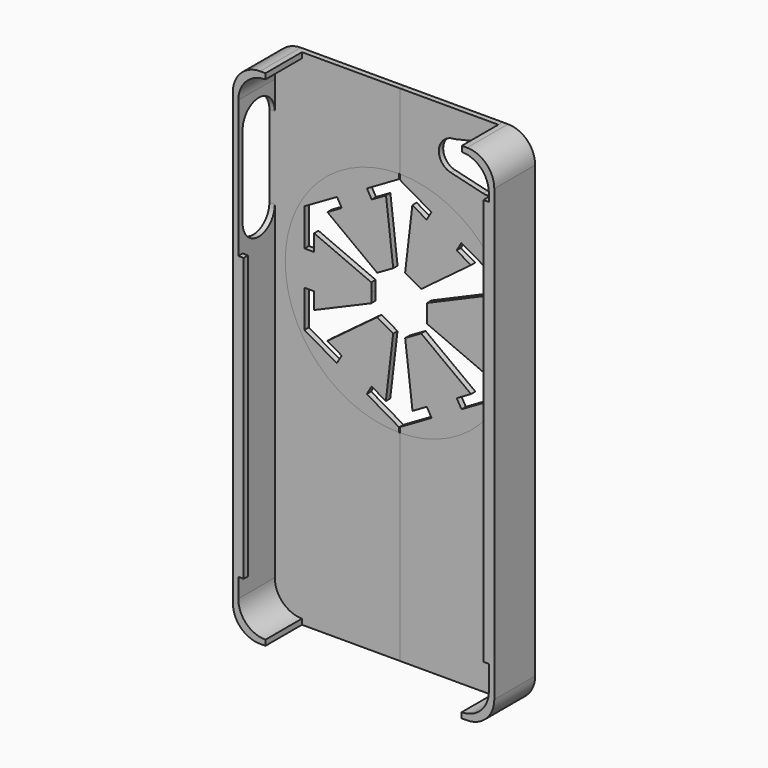
from build123d import *

# Parameters (mm, degrees)
F1_DEPTH  = 1.27
F2_DEPTH  = 11.938
F4_DEPTH  = 25.4
F5_DEPTH  = 1.27
F6_DEPTH  = 1.27
F7_W      = 1.27
F7_H      = 66
F8_DEPTH  = 1.27
F9_W      = 1.27
F9_H      = 95
F10_DEPTH = 1.27


# Not quite as in the source:
# - ends of sketch curves that miss each other by under 0.0002 mm in the source are joined


with BuildPart() as f1:
    # F0 (on Front) → F1 (new body)
    with BuildSketch(Plane.XZ):
        with BuildLine():
            ThreePointArc((-68.7733714747, 62.7475070371), (-73.2634995352, 60.8876350976), (-75.1233714747, 56.3975070371))
            Line((-75.1233714747, 56.3975070371), (-75.1233714747, -46.1422929629))
            ThreePointArc((-75.1233714747, -46.1422929629), (-73.2634995352, -50.6324210235), (-68.7733714747, -52.4922929629))
            Line((-68.7733714747, -52.4922929629), (-68.7733714747, -53.7622929629))
            Line((-68.7733714747, -53.7622929629), (-45.83683555, -53.7622929629))
            Line((-45.83683555, -53.7622929629), (-45.83683555, -6.8455746123))
            ThreePointArc((-45.83683555, -6.8455746123), (-45.9503157475, -6.8463001174), (-46.0637980065, -6.8465419539))
            ThreePointArc((-46.0637980065, -6.8465419539), (-64.8987750617, 0.95958485), (-72.689796607, 19.800815161))
            ThreePointArc((-72.689796607, 19.800815161), (-64.8836783627, 38.6144422615), (-46.0637980065, 46.4054723665))
            ThreePointArc((-46.0637980065, 46.4054723665), (-45.9503157475, 46.4052305299), (-45.83683555, 46.4045050248))
            Line((-45.83683555, 46.4045050248), (-45.83683555, 64.0175070371))
            Line((-45.83683555, 64.0175070371), (-68.7733714747, 64.0175070371))
            Line((-68.7733714747, 64.0175070371), (-68.7733714747, 62.7475070371))
        make_face()
    extrude(amount=F1_DEPTH)

    # F0 (on Front) → F2 (join)
    with BuildSketch(Plane.XZ):
        with BuildLine():
            Line((-75.1233714747, -46.1422929629), (-75.1233714747, 56.3975070371))
            ThreePointArc((-75.1233714747, 56.3975070371), (-73.2634995352, 60.8876350976), (-68.7733714747, 62.7475070371))
            Line((-68.7733714747, 62.7475070371), (-68.7733714747, 64.0175070371))
            Line((-68.7733714747, 64.0175070371), (-70.0433714747, 64.0175070371))
            ThreePointArc((-70.0433714747, 64.0175070371), (-74.5334995352, 62.1576350976), (-76.3933714747, 57.6675070371))
            Line((-76.3933714747, 57.6675070371), (-76.3933714747, -47.4122929629))
            ThreePointArc((-76.3933714747, -47.4122929629), (-74.5334995352, -51.9024210235), (-70.0433714747, -53.7622929629))
            Line((-70.0433714747, -53.7622929629), (-68.7733714747, -53.7622929629))
            Line((-68.7733714747, -53.7622929629), (-68.7733714747, -52.4922929629))
            ThreePointArc((-68.7733714747, -52.4922929629), (-73.2634995352, -50.6324210235), (-75.1233714747, -46.1422929629))
        make_face()
    extrude(amount=F2_DEPTH)

    # F3 (on face) → F4 (cut)
    with BuildSketch(Plane(origin=(-76.3933714747, 0, 0), x_dir=(0, -1, 0), z_dir=(-1, 0, 0))):
        with BuildLine():
            Line((10.668, 30.6165070371), (10.668, 49.7935070371))
            ThreePointArc((10.668, 49.7935070371), (5.969, 45.0945070371), (1.27, 49.7935070371))
            Line((1.27, 49.7935070371), (1.27, 30.6165070371))
            ThreePointArc((1.27, 30.6165070371), (5.969, 35.3155070371), (10.668, 30.6165070371))
        make_face()
        with BuildLine():
            ThreePointArc((1.27, 49.7935070371), (5.969, 45.0945070371), (10.668, 49.7935070371))
            ThreePointArc((10.668, 49.7935070371), (5.969, 54.4925070371), (1.27, 49.7935070371))
        make_face()
        with BuildLine():
            ThreePointArc((1.27, 30.6165070371), (5.969, 25.9175070371), (10.668, 30.6165070371))
            ThreePointArc((10.668, 30.6165070371), (5.969, 35.3155070371), (1.27, 30.6165070371))
        make_face()
    extrude(amount=-F4_DEPTH, mode=Mode.SUBTRACT)

    # F7 (on face) → F8 (join)
    with BuildSketch(Plane.YZ.offset(-75.1233714747)):
        with Locations((-11.303, -8.6227470934)):
            Rectangle(F7_W, F7_H)
    extrude(amount=F8_DEPTH)


with BuildPart() as f2:
    # F0 (on Front) → F2, piece 2 (new body)
    with BuildSketch(Plane.XZ):
        with BuildLine():
            Line((-21.6563714747, 64.0175070371), (-22.9002996252, 64.0175070371))
            Line((-22.9002996252, 64.0175070371), (-22.9002996252, 62.7475070371))
            ThreePointArc((-22.9002996252, 62.7475070371), (-18.4270350656, 60.8784613489), (-16.5763714747, 56.3975605602))
            Line((-16.5763714747, 56.3975605602), (-16.5763714747, -46.1422929629))
            ThreePointArc((-16.5763714747, -46.1422929629), (-18.4362434142, -50.6324210235), (-22.9263714747, -52.4922929629))
            Line((-22.9263714747, -52.4922929629), (-22.9263714747, -53.7622929629))
            Line((-22.9263714747, -53.7622929629), (-21.6563714747, -53.7622929629))
            ThreePointArc((-21.6563714747, -53.7622929629), (-17.1662434142, -51.9024210235), (-15.3063714747, -47.4122929629))
            Line((-15.3063714747, -47.4122929629), (-15.3063714747, 57.6675070371))
            ThreePointArc((-15.3063714747, 57.6675070371), (-17.1662434142, 62.1576350976), (-21.6563714747, 64.0175070371))
        make_face()
    extrude(amount=F2_DEPTH)

    # F9 (on face) → F10 (join)
    with BuildSketch(Plane(origin=(-16.5763714747, 0, 0), x_dir=(0, -1, 0), z_dir=(-1, 0, 0))):
        with Locations((11.303, 7.0158497989)):
            Rectangle(F9_W, F9_H)
    extrude(amount=F10_DEPTH)


with BuildPart() as f5:
    # F0 (on Front) → F5 (new body)
    with BuildSketch(Plane.XZ):
        with BuildLine():
            Line((-22.9002996252, 64.0175070371), (-45.83683555, 64.0175070371))
            Line((-45.83683555, 64.0175070371), (-45.83683555, 46.4045050248))
            ThreePointArc((-45.83683555, 46.4045050248), (-27.1638123458, 38.534059292), (-19.437799406, 19.800815161))
            ThreePointArc((-19.437799406, 19.800815161), (-19.4377929862, 19.7901401845), (-19.4377908463, 19.7794652063))
            ThreePointArc((-19.4377908463, 19.7794652063), (-27.1562947169, 1.0324500665), (-45.83683555, -6.8455746123))
            Line((-45.83683555, -6.8455746123), (-45.83683555, -53.7622929629))
            Line((-45.83683555, -53.7622929629), (-22.9263714747, -53.7622929629))
            Line((-22.9263714747, -53.7622929629), (-22.9263714747, -52.4922929629))
            ThreePointArc((-22.9263714747, -52.4922929629), (-18.4362434142, -50.6324210235), (-16.5763714747, -46.1422929629))
            Line((-16.5763714747, -46.1422929629), (-16.5763714747, 56.3975605602))
            ThreePointArc((-16.5763714747, 56.3975605602), (-18.4270350656, 60.8784613489), (-22.9002996252, 62.7475070371))
            Line((-22.9002996252, 62.7475070371), (-22.9002996252, 64.0175070371))
        make_face()
        with BuildLine():
            ThreePointArc((-25.2361353487, 59.5725070371), (-21.3578216202, 57.9660568916), (-19.7513714747, 54.0877431631))
            ThreePointArc((-19.7513714747, 54.0877431631), (-21.8412711567, 49.7798977769), (-26.5183106895, 48.7549520413))
            Line((-26.5183106895, 48.7549520413), (-34.0138568088, 50.5571235836))
            ThreePointArc((-34.0138568088, 50.5571235836), (-36.7709747399, 54.5151516939), (-33.1649817526, 57.7189775918))
            Line((-33.1649817526, 57.7189775918), (-27.6676093993, 59.0041004217))
            ThreePointArc((-27.6676093993, 59.0041004217), (-26.4846496797, 59.4285152719), (-25.2361353487, 59.5725070371))
        make_face(mode=Mode.SUBTRACT)
    extrude(amount=F5_DEPTH)


with BuildPart() as f6:
    # F0 (on Front) → F6 (new body)
    with BuildSketch(Plane.XZ):
        with BuildLine():
            ThreePointArc((-19.437799406, 19.800815161), (-27.1638123458, 38.534059292), (-45.83683555, 46.4045050248))
            Line((-45.83683555, 46.4045050248), (-45.83683555, 45.1567237107))
            Line((-45.83683555, 45.1567237107), (-38.5324436739, 40.9395310947))
            Line((-38.5324436739, 40.9395310947), (-31.5334607695, 36.8986664309))
            Line((-31.5334607695, 36.8986664309), (-23.972966235, 32.5336128762))
            Line((-23.972966235, 32.5336128762), (-23.972966235, 23.8371539736))
            Line((-23.972966235, 23.8371539736), (-23.972966235, 19.8148920808))
            Line((-23.972966235, 19.8148920808), (-23.972966235, 19.7971786549))
            Line((-23.972966235, 19.7971786549), (-19.437799406, 19.800815161))
        make_face()
        with BuildLine():
            Line((-45.83683555, -5.6209802107), (-45.83683555, -6.8455746123))
            ThreePointArc((-45.83683555, -6.8455746123), (-27.1562947169, 1.0324500665), (-19.4377908463, 19.7794652063))
            ThreePointArc((-19.4377908463, 19.7794652063), (-19.4377929862, 19.7901401845), (-19.437799406, 19.800815161))
            Line((-19.437799406, 19.800815161), (-23.972966235, 19.7971786549))
            Line((-23.972966235, 19.7971786549), (-23.972966235, 19.7794652063))
            Line((-23.972966235, 19.7794652063), (-23.9664873618, 15.7572085313))
            Line((-23.9664873618, 15.7572085313), (-23.9525409264, 7.0607608116))
            Line((-23.9525409264, 7.0607608116), (-31.5060255403, 2.6835881708))
            Line((-31.5060255403, 2.6835881708), (-38.4985191452, -1.3684955049))
            Line((-38.4985191452, -1.3684955049), (-45.83683555, -5.6209802107))
        make_face()
        Polygon((-31.5334607695, 36.8986664309), (-38.5324436739, 40.9395310947), (-39.6432602587, 39.0119725608), (-32.6425828079, 34.9776107085), align=None)
        Polygon((-23.972966235, 19.7794652063), (-23.972966235, 19.7971786549), (-26.1944497484, 19.7953973669), (-26.1912103118, 15.7554246458), (-23.9664873618, 15.7572085313), align=None)
        Polygon((-26.1944497484, 19.7953973669), (-23.972966235, 19.7971786549), (-23.972966235, 19.8148920808), (-23.972966235, 23.8371539736), (-26.1976891851, 23.835370088), align=None)
        Polygon((-39.6124255104, 0.5572791435), (-38.4985191452, -1.3684955049), (-31.5060255403, 2.6835881708), (-32.6182269329, 4.6028627334), align=None)
        Polygon((-39.6432602587, 39.0119725608), (-42.988080594, 40.9395310947), (-44.6731523984, 26.5053643083), (-40.9343213249, 24.3467491815), (-29.2977624726, 33.0500521746), (-32.6425828079, 34.9776107085), align=None)
        Polygon((-26.1912103118, 15.7554246458), (-26.1944497484, 19.7953973669), (-39.5436757168, 19.7846933413), (-39.5436757168, 19.7794652063), (-39.5402223489, 17.6313091186), (-26.1881148018, 11.8949459974), align=None)
        Polygon((-39.5436757168, 19.7846933413), (-26.1944497484, 19.7953973669), (-26.1976891851, 23.835370088), (-26.200784695, 27.6958487364), (-39.5436757168, 21.938080333), (-39.5436757168, 19.7899214696), align=None)
        Polygon((-44.6623679209, 13.0558049194), (-42.9541503357, -1.375640971), (-39.6124255104, 0.5572791435), (-32.6182269329, 4.6028627334), (-29.2765021076, 6.5357828479), (-40.9270034074, 15.2204132012), align=None)
    extrude(amount=F6_DEPTH)


with BuildPart() as f6b:
    # F0 (on Front) → F6, piece 2 (new body)
    with BuildSketch(Plane.XZ):
        with BuildLine():
            Line((-46.0637980065, 45.2877605461), (-46.0637980065, 46.4054723665))
            ThreePointArc((-46.0637980065, 46.4054723665), (-64.8836783627, 38.6144422615), (-72.689796607, 19.800815161))
            Line((-72.689796607, 19.800815161), (-68.154629778, 19.7971786549))
            Line((-68.154629778, 19.7971786549), (-68.1546013711, 19.8148920808))
            Line((-68.1546013711, 19.8148920808), (-68.154629778, 23.8371539736))
            Line((-68.154629778, 23.8371539736), (-68.154629778, 32.5336128762))
            Line((-68.154629778, 32.5336128762), (-60.5941352435, 36.8986664309))
            Line((-60.5941352435, 36.8986664309), (-53.5951523391, 40.9395310947))
            Line((-53.5951523391, 40.9395310947), (-46.0637980065, 45.2877605461))
        make_face()
        with BuildLine():
            ThreePointArc((-72.689796607, 19.800815161), (-64.8987750617, 0.95958485), (-46.0637980065, -6.8465419539))
            Line((-46.0637980065, -6.8465419539), (-46.0637980065, -5.7525028001))
            Line((-46.0637980065, -5.7525028001), (-46.1047054376, -5.7287973321))
            Line((-46.1047054376, -5.7287973321), (-53.6290768678, -1.3684955049))
            Line((-53.6290768678, -1.3684955049), (-60.6215704726, 2.6835881708))
            Line((-60.6215704726, 2.6835881708), (-68.1750550866, 7.0607608116))
            Line((-68.1750550866, 7.0607608116), (-68.1611086512, 15.7572085313))
            Line((-68.1611086512, 15.7572085313), (-68.1546581848, 19.7794652518))
            Line((-68.1546581848, 19.7794652518), (-68.154629778, 19.7971786549))
            Line((-68.154629778, 19.7971786549), (-72.689796607, 19.800815161))
        make_face()
        Polygon((-52.4843357543, 39.0119725608), (-53.5951523391, 40.9395310947), (-60.5941352435, 36.8986664309), (-59.4850132051, 34.9776107085), align=None)
        Polygon((-65.9331462645, 19.7953973669), (-68.154629778, 19.7971786549), (-68.1546581848, 19.7794652518), (-68.1611086512, 15.7572085313), (-65.9363857011, 15.7554246458), align=None)
        Polygon((-68.1546013711, 19.8148920808), (-68.154629778, 19.7971786549), (-65.9331462645, 19.7953973669), (-65.9299068279, 23.835370088), (-68.154629778, 23.8371539736), align=None)
        Polygon((-47.4544436145, 26.5053643083), (-49.139515419, 40.9395310947), (-52.4843357543, 39.0119725608), (-59.4850132051, 34.9776107085), (-62.8298335403, 33.0500521746), (-51.1932746881, 24.3467491815), align=None)
        Polygon((-52.5839202961, 19.7846933413), (-65.9331462645, 19.7953973669), (-65.9363857011, 15.7554246458), (-65.9394812111, 11.8949459974), (-52.5873736641, 17.6313091186), (-52.5839286804, 19.7794652197), align=None)
        Polygon((-65.9299068279, 23.835370088), (-65.9331462645, 19.7953973669), (-52.5839202961, 19.7846933413), (-52.5839202961, 19.7899214696), (-52.5839202961, 21.938080333), (-65.9268113179, 27.6958487364), align=None)
        Polygon((-60.6215704726, 2.6835881708), (-53.6290768678, -1.3684955049), (-52.5151705026, 0.5572791435), (-59.5093690801, 4.6028627334), align=None)
        Polygon((-49.1734456773, -1.375640971), (-47.4652280921, 13.0558049194), (-51.2005926056, 15.2204132012), (-62.8510939054, 6.5357828479), (-59.5093690801, 4.6028627334), (-52.5151705026, 0.5572791435), align=None)
    extrude(amount=F6_DEPTH)


solid = Compound([f1.part, f2.part, f5.part, f6.part, f6b.part])
